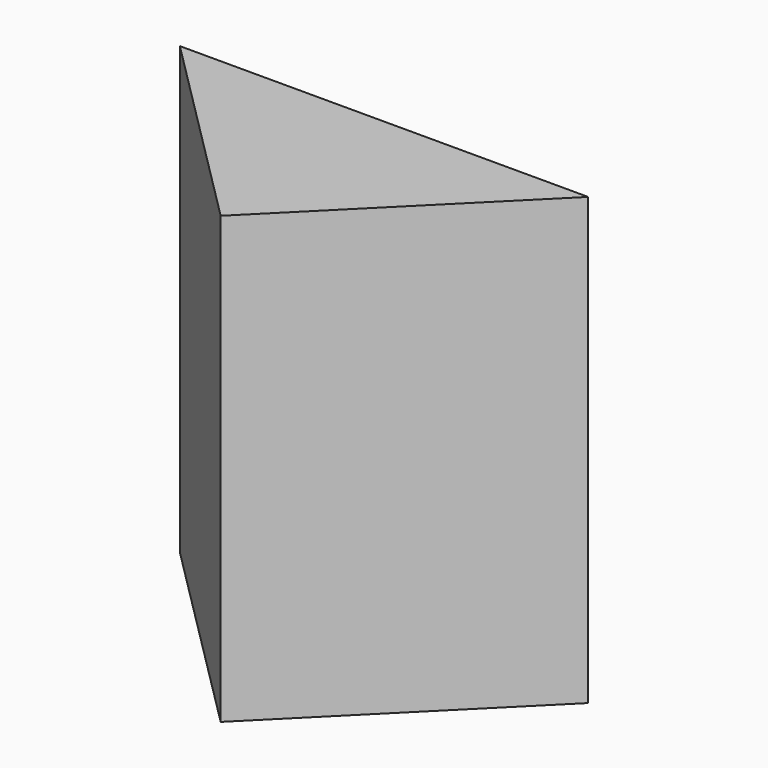
from build123d import *

# Parameters (mm, degrees)
F0_W        = 91.1898128688
F0_H        = 99.5126962662
F1_DEPTH    = 50.8
F2_T1_DEPTH = 360.7956878435


# Not quite as in the source:
# - a fillet or chamfer that OpenCascade refuses, or shapes differently, is made with other operations: its cross-section is extruded or revolved along the edge and cut away or added


with BuildPart() as f1:
    # F0 (on Front) → F1 (new body)
    with BuildSketch(Plane.XZ):
        with Locations((6.69449009, -1.6283914447)):
            Rectangle(F0_W, F0_H)
    extrude(amount=F1_DEPTH)

    # F2: chamfer of 50.8 on 2 edges, made by hand

    # F2_s2 → F2_t1 (cut)
    with BuildSketch(Plane.XY.offset(-182.0262353664)):
        Polygon((-38.9004163444, 0), (11.8995836556, -50.8), (-38.9004163444, -50.8), align=None)
        Polygon((52.2893965244, 0), (1.4893965244, -50.8), (52.2893965244, -50.8), align=None)
    extrude(amount=F2_T1_DEPTH, mode=Mode.SUBTRACT)


solid = f1.part
